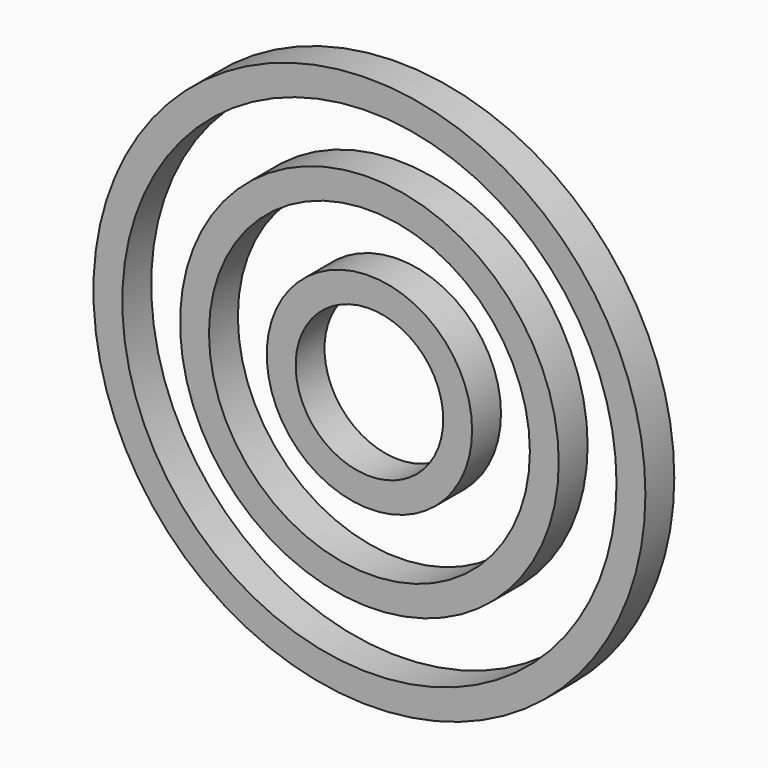
from build123d import *

# Parameters (mm, degrees)
F0_R     = 191.1000013351
F0_R_2   = 171.0999992129
F1_DEPTH = 25
F0_R_3   = 71.1000000685
F0_R_4   = 51.0999997705
F0_R_5   = 131.0999962257
F0_R_6   = 111.1000000685


with BuildPart() as f1:
    # F0 (on Front) → F1 (new body)
    with BuildSketch(Plane.XZ):
        Circle(F0_R)
        Circle(F0_R_2, mode=Mode.SUBTRACT)
    extrude(amount=F1_DEPTH)


with BuildPart() as f1b:
    # F0 (on Front) → F1, piece 2 (new body)
    with BuildSketch(Plane.XZ):
        Circle(F0_R_3)
        Circle(F0_R_4, mode=Mode.SUBTRACT)
    extrude(amount=F1_DEPTH)


with BuildPart() as f1c:
    # F0 (on Front) → F1, piece 3 (new body)
    with BuildSketch(Plane.XZ):
        Circle(F0_R_5)
        Circle(F0_R_6, mode=Mode.SUBTRACT)
    extrude(amount=F1_DEPTH)


solid = Compound([f1.part, f1b.part, f1c.part])
